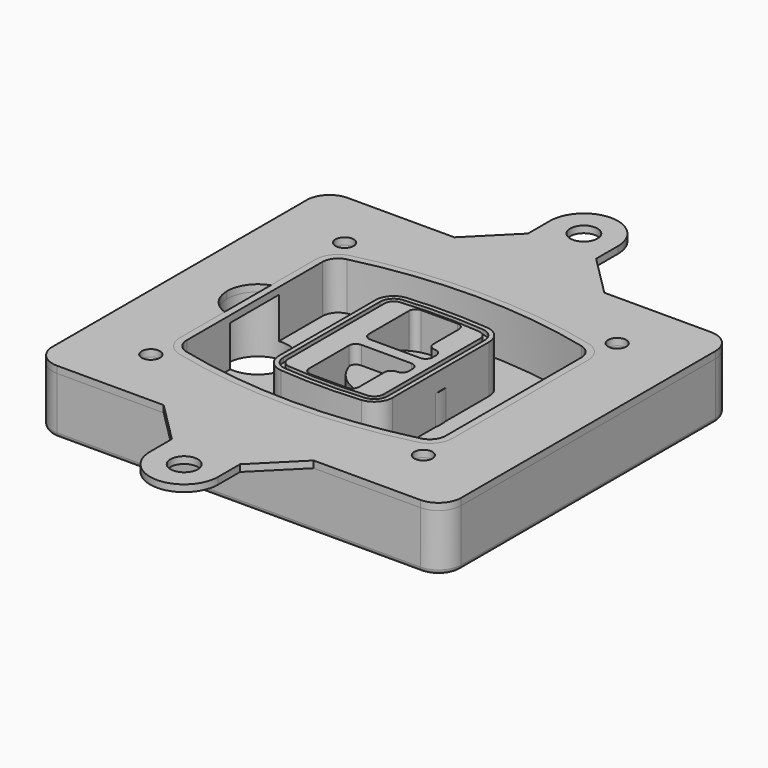
from build123d import *

# Parameters (mm, degrees)
F0_R      = 4
F1_DEPTH  = 25
F2_DEPTH  = 3
F3_DEPTH  = 18
F5_DEPTH  = 21
F6_DEPTH  = 2
F8_DEPTH  = 20
F9_DEPTH  = 16
F10_DEPTH = 25
F7_R      = 6
F7_R_2    = 4
F11_DEPTH = 6
F13_DEPTH = 9
F15_R     = 2
F16_R     = 6
F16_R_2   = 4
F17_DEPTH = 3


# Not quite as in the source:
# - a feature of the source that left no trace in its solid (it failed there, or was rolled back) is left out
# - a feature names something its author has since deleted; it is built from what else it names


with BuildPart() as f1:
    # F0 (on Top) → F1 (new body)
    with BuildSketch(Plane.XY):
        with BuildLine():
            ThreePointArc((-90, -70), (-87.0710678119, -77.0710678119), (-80, -80))
            Line((-80, -80), (80, -80))
            ThreePointArc((80, -80), (87.0710678119, -77.0710678119), (90, -70))
            Line((90, -70), (90, 70))
            ThreePointArc((90, 70), (87.0710678119, 77.0710678119), (80, 80))
            Line((80, 80), (-80, 80))
            ThreePointArc((-80, 80), (-87.0710678119, 77.0710678119), (-90, 70))
            Line((-90, 70), (-90, -70))
        make_face()
        with Locations((-60, -53.3333333333)):
            Circle(F0_R, mode=Mode.SUBTRACT)
        with Locations((60, -53.3333333333)):
            Circle(F0_R, mode=Mode.SUBTRACT)
        with Locations((-60, 53.3333333333)):
            Circle(F0_R, mode=Mode.SUBTRACT)
        with BuildLine():
            ThreePointArc((-64, 37.2990447398), (-61.0143011354, 45.9411029726), (-53.3306899286, 50.8970778549))
            ThreePointArc((-53.3306899286, 50.8970778549), (0, 57.3333333333), (53.3306899286, 50.8970778549))
            ThreePointArc((53.3306899286, 50.8970778549), (61.0143011354, 45.9411029726), (64, 37.2990447398))
            Line((64, 37.2990447398), (64, -37.2990447398))
            ThreePointArc((64, -37.2990447398), (61.0143011354, -45.9411029726), (53.3306899286, -50.8970778549))
            ThreePointArc((53.3306899286, -50.8970778549), (0, -57.3333333333), (-53.3306899286, -50.8970778549))
            ThreePointArc((-53.3306899286, -50.8970778549), (-61.0143011354, -45.9411029726), (-64, -37.2990447398))
            Line((-64, -37.2990447398), (-64, 37.2990447398))
        make_face(mode=Mode.SUBTRACT)
        with Locations((60, 53.3333333333)):
            Circle(F0_R, mode=Mode.SUBTRACT)
        with BuildLine():
            ThreePointArc((53.3306899286, 50.8970778549), (0, 57.3333333333), (-53.3306899286, 50.8970778549))
            ThreePointArc((-53.3306899286, 50.8970778549), (-61.0143011354, 45.9411029726), (-64, 37.2990447398))
            Line((-64, 37.2990447398), (-64, -37.2990447398))
            ThreePointArc((-64, -37.2990447398), (-61.0143011354, -45.9411029726), (-53.3306899286, -50.8970778549))
            ThreePointArc((-53.3306899286, -50.8970778549), (0, -57.3333333333), (53.3306899286, -50.8970778549))
            ThreePointArc((53.3306899286, -50.8970778549), (61.0143011354, -45.9411029726), (64, -37.2990447398))
            Line((64, -37.2990447398), (64, 37.2990447398))
            ThreePointArc((64, 37.2990447398), (61.0143011354, 45.9411029726), (53.3306899286, 50.8970778549))
        make_face()
        with BuildLine():
            Line((-60, -37.2990447398), (-60, 37.2990447398))
            ThreePointArc((-60, 37.2990447398), (-57.8673579538, 43.4719434775), (-52.3790642347, 47.0119255363))
            ThreePointArc((-52.3790642347, 47.0119255363), (0, 53.3333333333), (52.3790642347, 47.0119255363))
            ThreePointArc((52.3790642347, 47.0119255363), (57.8673579538, 43.4719434775), (60, 37.2990447398))
            Line((60, 37.2990447398), (60, -37.2990447398))
            ThreePointArc((60, -37.2990447398), (57.8673579538, -43.4719434775), (52.3790642347, -47.0119255363))
            ThreePointArc((52.3790642347, -47.0119255363), (0, -53.3333333333), (-52.3790642347, -47.0119255363))
            ThreePointArc((-52.3790642347, -47.0119255363), (-57.8673579538, -43.4719434775), (-60, -37.2990447398))
        make_face(mode=Mode.SUBTRACT)
        with BuildLine():
            ThreePointArc((-52.3790642347, 47.0119255363), (-57.8673579538, 43.4719434775), (-60, 37.2990447398))
            Line((-60, 37.2990447398), (-60, -37.2990447398))
            ThreePointArc((-60, -37.2990447398), (-57.8673579538, -43.4719434775), (-52.3790642347, -47.0119255363))
            ThreePointArc((-52.3790642347, -47.0119255363), (0, -53.3333333333), (52.3790642347, -47.0119255363))
            ThreePointArc((52.3790642347, -47.0119255363), (57.8673579538, -43.4719434775), (60, -37.2990447398))
            Line((60, -37.2990447398), (60, 37.2990447398))
            ThreePointArc((60, 37.2990447398), (57.8673579538, 43.4719434775), (52.3790642347, 47.0119255363))
            ThreePointArc((52.3790642347, 47.0119255363), (0, 53.3333333333), (-52.3790642347, 47.0119255363))
        make_face()
        with BuildLine():
            ThreePointArc((51.6653449643, 44.0980612973), (55.5071505677, 41.6200738562), (57, 37.2990447398))
            Line((57, 37.2990447398), (57, -37.2990447398))
            ThreePointArc((57, -37.2990447398), (55.5071505677, -41.6200738562), (51.6653449643, -44.0980612973))
            ThreePointArc((51.6653449643, -44.0980612973), (0, -50.3333333333), (-51.6653449643, -44.0980612973))
            ThreePointArc((-51.6653449643, -44.0980612973), (-55.5071505677, -41.6200738562), (-57, -37.2990447398))
            Line((-57, -37.2990447398), (-57, 37.2990447398))
            ThreePointArc((-57, 37.2990447398), (-55.5071505677, 41.6200738562), (-51.6653449643, 44.0980612973))
            ThreePointArc((-51.6653449643, 44.0980612973), (0, 50.3333333333), (51.6653449643, 44.0980612973))
        make_face(mode=Mode.SUBTRACT)
        with BuildLine():
            Line((57, -37.2990447398), (57, 37.2990447398))
            ThreePointArc((57, 37.2990447398), (55.5071505677, 41.6200738562), (51.6653449643, 44.0980612973))
            ThreePointArc((51.6653449643, 44.0980612973), (0, 50.3333333333), (-51.6653449643, 44.0980612973))
            ThreePointArc((-51.6653449643, 44.0980612973), (-55.5071505677, 41.6200738562), (-57, 37.2990447398))
            Line((-57, 37.2990447398), (-57, -37.2990447398))
            ThreePointArc((-57, -37.2990447398), (-55.5071505677, -41.6200738562), (-51.6653449643, -44.0980612973))
            ThreePointArc((-51.6653449643, -44.0980612973), (0, -50.3333333333), (51.6653449643, -44.0980612973))
            ThreePointArc((51.6653449643, -44.0980612973), (55.5071505677, -41.6200738562), (57, -37.2990447398))
        make_face()
    extrude(amount=-F1_DEPTH)

    # F0 (on Top) → F2 (join)
    with BuildSketch(Plane.XY):
        with BuildLine():
            ThreePointArc((-52.3790642347, 47.0119255363), (-57.8673579538, 43.4719434775), (-60, 37.2990447398))
            Line((-60, 37.2990447398), (-60, -37.2990447398))
            ThreePointArc((-60, -37.2990447398), (-57.8673579538, -43.4719434775), (-52.3790642347, -47.0119255363))
            ThreePointArc((-52.3790642347, -47.0119255363), (0, -53.3333333333), (52.3790642347, -47.0119255363))
            ThreePointArc((52.3790642347, -47.0119255363), (57.8673579538, -43.4719434775), (60, -37.2990447398))
            Line((60, -37.2990447398), (60, 37.2990447398))
            ThreePointArc((60, 37.2990447398), (57.8673579538, 43.4719434775), (52.3790642347, 47.0119255363))
            ThreePointArc((52.3790642347, 47.0119255363), (0, 53.3333333333), (-52.3790642347, 47.0119255363))
        make_face()
        with BuildLine():
            ThreePointArc((51.6653449643, 44.0980612973), (55.5071505677, 41.6200738562), (57, 37.2990447398))
            Line((57, 37.2990447398), (57, -37.2990447398))
            ThreePointArc((57, -37.2990447398), (55.5071505677, -41.6200738562), (51.6653449643, -44.0980612973))
            ThreePointArc((51.6653449643, -44.0980612973), (0, -50.3333333333), (-51.6653449643, -44.0980612973))
            ThreePointArc((-51.6653449643, -44.0980612973), (-55.5071505677, -41.6200738562), (-57, -37.2990447398))
            Line((-57, -37.2990447398), (-57, 37.2990447398))
            ThreePointArc((-57, 37.2990447398), (-55.5071505677, 41.6200738562), (-51.6653449643, 44.0980612973))
            ThreePointArc((-51.6653449643, 44.0980612973), (0, 50.3333333333), (51.6653449643, 44.0980612973))
        make_face(mode=Mode.SUBTRACT)
    extrude(amount=F2_DEPTH)

    # F0 (on Top) → F3 (cut)
    with BuildSketch(Plane.XY):
        with BuildLine():
            Line((57, -37.2990447398), (57, 37.2990447398))
            ThreePointArc((57, 37.2990447398), (55.5071505677, 41.6200738562), (51.6653449643, 44.0980612973))
            ThreePointArc((51.6653449643, 44.0980612973), (0, 50.3333333333), (-51.6653449643, 44.0980612973))
            ThreePointArc((-51.6653449643, 44.0980612973), (-55.5071505677, 41.6200738562), (-57, 37.2990447398))
            Line((-57, 37.2990447398), (-57, -37.2990447398))
            ThreePointArc((-57, -37.2990447398), (-55.5071505677, -41.6200738562), (-51.6653449643, -44.0980612973))
            ThreePointArc((-51.6653449643, -44.0980612973), (0, -50.3333333333), (51.6653449643, -44.0980612973))
            ThreePointArc((51.6653449643, -44.0980612973), (55.5071505677, -41.6200738562), (57, -37.2990447398))
        make_face()
    extrude(amount=-F3_DEPTH, mode=Mode.SUBTRACT)

    # F4 (on face) → F5 (join, through all)
    with BuildSketch(Plane.XY.offset(3)):
        with BuildLine():
            ThreePointArc((-25, -26.587695628), (-22.8992979869, -31.9912392117), (-17.7004291845, -34.5569740744))
            ThreePointArc((-17.7004291845, -34.5569740744), (0, -35.3333333333), (17.7004291845, -34.5569740744))
            ThreePointArc((17.7004291845, -34.5569740744), (22.8992979869, -31.9912392117), (25, -26.587695628))
            Line((25, -26.587695628), (25, 26.587695628))
            ThreePointArc((25, 26.587695628), (22.8992979869, 31.9912392117), (17.7004291845, 34.5569740744))
            ThreePointArc((17.7004291845, 34.5569740744), (0, 35.3333333333), (-17.7004291845, 34.5569740744))
            ThreePointArc((-17.7004291845, 34.5569740744), (-22.8992979869, 31.9912392117), (-25, 26.587695628))
            Line((-25, 26.587695628), (-25, -26.587695628))
        make_face()
        with BuildLine():
            ThreePointArc((17.5253218884, 32.5646544628), (21.4244734902, 30.6403533158), (23, 26.587695628))
            Line((23, 26.587695628), (23, -26.587695628))
            ThreePointArc((23, -26.587695628), (21.4244734902, -30.6403533158), (17.5253218884, -32.5646544628))
            ThreePointArc((17.5253218884, -32.5646544628), (0, -33.3333333333), (-17.5253218884, -32.5646544628))
            ThreePointArc((-17.5253218884, -32.5646544628), (-21.4244734902, -30.6403533158), (-23, -26.587695628))
            Line((-23, -26.587695628), (-23, 26.587695628))
            ThreePointArc((-23, 26.587695628), (-21.4244734902, 30.6403533158), (-17.5253218884, 32.5646544628))
            ThreePointArc((-17.5253218884, 32.5646544628), (0, 33.3333333333), (17.5253218884, 32.5646544628))
        make_face(mode=Mode.SUBTRACT)
        with BuildLine():
            Line((23, -26.587695628), (23, 26.587695628))
            ThreePointArc((23, 26.587695628), (21.4244734902, 30.6403533158), (17.5253218884, 32.5646544628))
            ThreePointArc((17.5253218884, 32.5646544628), (0, 33.3333333333), (-17.5253218884, 32.5646544628))
            ThreePointArc((-17.5253218884, 32.5646544628), (-21.4244734902, 30.6403533158), (-23, 26.587695628))
            Line((-23, 26.587695628), (-23, -26.587695628))
            ThreePointArc((-23, -26.587695628), (-21.4244734902, -30.6403533158), (-17.5253218884, -32.5646544628))
            ThreePointArc((-17.5253218884, -32.5646544628), (0, -33.3333333333), (17.5253218884, -32.5646544628))
            ThreePointArc((17.5253218884, -32.5646544628), (21.4244734902, -30.6403533158), (23, -26.587695628))
        make_face()
        with BuildLine():
            ThreePointArc((17.3502145923, 30.5723348512), (19.9496489934, 29.2894674198), (21, 26.587695628))
            Line((21, 26.587695628), (21, -26.587695628))
            ThreePointArc((21, -26.587695628), (19.9496489934, -29.2894674198), (17.3502145923, -30.5723348512))
            ThreePointArc((17.3502145923, -30.5723348512), (0, -31.3333333333), (-17.3502145923, -30.5723348512))
            ThreePointArc((-17.3502145923, -30.5723348512), (-19.9496489934, -29.2894674198), (-21, -26.587695628))
            Line((-21, -26.587695628), (-21, 26.587695628))
            ThreePointArc((-21, 26.587695628), (-19.9496489934, 29.2894674198), (-17.3502145923, 30.5723348512))
            ThreePointArc((-17.3502145923, 30.5723348512), (0, 31.3333333333), (17.3502145923, 30.5723348512))
        make_face(mode=Mode.SUBTRACT)
        with BuildLine():
            Line((21, -26.587695628), (21, 26.587695628))
            ThreePointArc((21, 26.587695628), (19.9496489934, 29.2894674198), (17.3502145923, 30.5723348512))
            ThreePointArc((17.3502145923, 30.5723348512), (0, 31.3333333333), (-17.3502145923, 30.5723348512))
            ThreePointArc((-17.3502145923, 30.5723348512), (-19.9496489934, 29.2894674198), (-21, 26.587695628))
            Line((-21, 26.587695628), (-21, -26.587695628))
            ThreePointArc((-21, -26.587695628), (-19.9496489934, -29.2894674198), (-17.3502145923, -30.5723348512))
            ThreePointArc((-17.3502145923, -30.5723348512), (0, -31.3333333333), (17.3502145923, -30.5723348512))
            ThreePointArc((17.3502145923, -30.5723348512), (19.9496489934, -29.2894674198), (21, -26.587695628))
        make_face()
        with BuildLine():
            Line((-8, -2.5), (14, -2.5))
            ThreePointArc((14, -2.5), (16.1213203436, -3.3786796564), (17, -5.5))
            Line((17, -5.5), (17, -7.5))
            ThreePointArc((17, -7.5), (16.1213203436, -9.6213203436), (14, -10.5))
            ThreePointArc((14, -10.5), (11.8786796564, -11.3786796564), (11, -13.5))
            Line((11, -13.5), (11, -27.5))
            ThreePointArc((11, -27.5), (10.1213203436, -29.6213203436), (8, -30.5))
            Line((8, -30.5), (-8, -30.5))
            ThreePointArc((-8, -30.5), (-10.1213203436, -29.6213203436), (-11, -27.5))
            Line((-11, -27.5), (-11, -5.5))
            ThreePointArc((-11, -5.5), (-10.1213203436, -3.3786796564), (-8, -2.5))
        make_face(mode=Mode.SUBTRACT)
        with BuildLine():
            ThreePointArc((-8, 2.5), (-10.1213203436, 3.3786796564), (-11, 5.5))
            Line((-11, 5.5), (-11, 27.5))
            ThreePointArc((-11, 27.5), (-10.1213203436, 29.6213203436), (-8, 30.5))
            Line((-8, 30.5), (8, 30.5))
            ThreePointArc((8, 30.5), (10.1213203436, 29.6213203436), (11, 27.5))
            Line((11, 27.5), (11, 13.5))
            ThreePointArc((11, 13.5), (11.8786796564, 11.3786796564), (14, 10.5))
            ThreePointArc((14, 10.5), (16.1213203436, 9.6213203436), (17, 7.5))
            Line((17, 7.5), (17, 5.5))
            ThreePointArc((17, 5.5), (16.1213203436, 3.3786796564), (14, 2.5))
            Line((14, 2.5), (-8, 2.5))
        make_face(mode=Mode.SUBTRACT)
    extrude(amount=-F5_DEPTH)

    # F4 (on face) → F6 (cut)
    with BuildSketch(Plane.XY.offset(3)):
        with BuildLine():
            Line((23, -26.587695628), (23, 26.587695628))
            ThreePointArc((23, 26.587695628), (21.4244734902, 30.6403533158), (17.5253218884, 32.5646544628))
            ThreePointArc((17.5253218884, 32.5646544628), (0, 33.3333333333), (-17.5253218884, 32.5646544628))
            ThreePointArc((-17.5253218884, 32.5646544628), (-21.4244734902, 30.6403533158), (-23, 26.587695628))
            Line((-23, 26.587695628), (-23, -26.587695628))
            ThreePointArc((-23, -26.587695628), (-21.4244734902, -30.6403533158), (-17.5253218884, -32.5646544628))
            ThreePointArc((-17.5253218884, -32.5646544628), (0, -33.3333333333), (17.5253218884, -32.5646544628))
            ThreePointArc((17.5253218884, -32.5646544628), (21.4244734902, -30.6403533158), (23, -26.587695628))
        make_face()
        with BuildLine():
            ThreePointArc((17.3502145923, 30.5723348512), (19.9496489934, 29.2894674198), (21, 26.587695628))
            Line((21, 26.587695628), (21, -26.587695628))
            ThreePointArc((21, -26.587695628), (19.9496489934, -29.2894674198), (17.3502145923, -30.5723348512))
            ThreePointArc((17.3502145923, -30.5723348512), (0, -31.3333333333), (-17.3502145923, -30.5723348512))
            ThreePointArc((-17.3502145923, -30.5723348512), (-19.9496489934, -29.2894674198), (-21, -26.587695628))
            Line((-21, -26.587695628), (-21, 26.587695628))
            ThreePointArc((-21, 26.587695628), (-19.9496489934, 29.2894674198), (-17.3502145923, 30.5723348512))
            ThreePointArc((-17.3502145923, 30.5723348512), (0, 31.3333333333), (17.3502145923, 30.5723348512))
        make_face(mode=Mode.SUBTRACT)
    extrude(amount=-F6_DEPTH, mode=Mode.SUBTRACT)

    # F7 (on face) → F8 (join)
    with BuildSketch(Plane(origin=(0, 0, -25), x_dir=(1, 0, 0), z_dir=(0, 0, -1))):
        with BuildLine():
            ThreePointArc((-6.71157564, 0), (6.7567035675, 13.4682792075), (20.224982775, 0))
            Line((20.224982775, 0), (25.224982775, 0))
            ThreePointArc((25.224982775, 0), (6.7567035675, 18.4682792075), (-11.71157564, 0))
            Line((-11.71157564, 0), (-6.71157564, 0))
        make_face()
        with BuildLine():
            Line((-6.71157564, 0), (20.224982775, 0))
            ThreePointArc((20.224982775, 0), (6.7567035675, 13.4682792075), (-6.71157564, 0))
        make_face()
        with BuildLine():
            ThreePointArc((-6.71157564, 0), (6.7567035675, -13.4682792075), (20.224982775, 0))
            Line((20.224982775, 0), (-6.71157564, 0))
        make_face()
        with BuildLine():
            Line((25.224982775, 0), (20.224982775, 0))
            ThreePointArc((20.224982775, 0), (6.7567035675, -13.4682792075), (-6.71157564, 0))
            Line((-6.71157564, 0), (-11.71157564, 0))
            ThreePointArc((-11.71157564, 0), (6.7567035675, -18.4682792075), (25.224982775, 0))
        make_face()
    extrude(amount=-F8_DEPTH)

    # F7 (on face) → F9 (cut)
    with BuildSketch(Plane(origin=(0, 0, -25), x_dir=(1, 0, 0), z_dir=(0, 0, -1))):
        with BuildLine():
            Line((-6.71157564, 0), (20.224982775, 0))
            ThreePointArc((20.224982775, 0), (6.7567035675, 13.4682792075), (-6.71157564, 0))
        make_face()
        with BuildLine():
            ThreePointArc((-6.71157564, 0), (6.7567035675, -13.4682792075), (20.224982775, 0))
            Line((20.224982775, 0), (-6.71157564, 0))
        make_face()
    extrude(amount=-F9_DEPTH, mode=Mode.SUBTRACT)

    # F7 (on face) → F10 (cut)
    with BuildSketch(Plane(origin=(0, 0, -25), x_dir=(1, 0, 0), z_dir=(0, 0, -1))):
        with BuildLine():
            Line((-69.0318229325, 0), (-42.0952645175, 0))
            ThreePointArc((-42.0952645175, 0), (-55.563543725, 13.4682792075), (-69.0318229325, 0))
        make_face()
        with BuildLine():
            ThreePointArc((-69.0318229325, 0), (-55.563543725, -13.4682792075), (-42.0952645175, 0))
            Line((-42.0952645175, 0), (-69.0318229325, 0))
        make_face()
    extrude(amount=-F10_DEPTH, mode=Mode.SUBTRACT)

    # F7 (on face) → F11 (cut)
    with BuildSketch(Plane(origin=(0, 0, -25), x_dir=(1, 0, 0), z_dir=(0, 0, -1))):
        with Locations((60, -53.3333333333)):
            Circle(F7_R)
        with Locations((60, -53.3333333333)):
            Circle(F7_R_2, mode=Mode.SUBTRACT)
        with Locations((-60, -53.3333333333)):
            Circle(F7_R)
        with Locations((-60, -53.3333333333)):
            Circle(F7_R_2, mode=Mode.SUBTRACT)
        with Locations((-60, 53.3333333333)):
            Circle(F7_R)
        with Locations((-60, 53.3333333333)):
            Circle(F7_R_2, mode=Mode.SUBTRACT)
        with Locations((60, 53.3333333333)):
            Circle(F7_R)
        with Locations((60, 53.3333333333)):
            Circle(F7_R_2, mode=Mode.SUBTRACT)
    extrude(amount=-F11_DEPTH, mode=Mode.SUBTRACT)

    # F12 (on face) → F13 (cut, through all)
    with BuildSketch(Plane(origin=(0, 0, -9), x_dir=(1, 0, 0), z_dir=(0, 0, -1))):
        with BuildLine():
            ThreePointArc((20.224982775, 0), (20.1663399806, 1.2554664788), (19.9909222755, 2.5))
            Line((19.9909222755, 2.5), (14, 2.5))
            ThreePointArc((14, 2.5), (16.1213203436, 3.3786796564), (17, 5.5))
            Line((17, 5.5), (17, 7.5))
            ThreePointArc((17, 7.5), (16.1213203436, 9.6213203436), (14, 10.5))
            ThreePointArc((14, 10.5), (12.1627255951, 11.1284134507), (11.0951631559, 12.750384826))
            ThreePointArc((11.0951631559, 12.750384826), (11.0476113807, 12.7664660322), (11, 12.7823698976))
            Line((11, 12.7823698976), (11, -12.7823698976))
            ThreePointArc((11, -12.7823698976), (11.0476113807, -12.7664660322), (11.0951631559, -12.750384826))
            ThreePointArc((11.0951631559, -12.750384826), (12.1627255951, -11.1284134507), (14, -10.5))
            ThreePointArc((14, -10.5), (16.1213203436, -9.6213203436), (17, -7.5))
            Line((17, -7.5), (17, -5.5))
            ThreePointArc((17, -5.5), (16.1213203436, -3.3786796564), (14, -2.5))
            Line((14, -2.5), (19.9909222755, -2.5))
            ThreePointArc((19.9909222755, -2.5), (20.1663399806, -1.2554664788), (20.224982775, 0))
        make_face()
    extrude(amount=F13_DEPTH, mode=Mode.SUBTRACT)

    # F15
    f15_edges = [f1.edges().sort_by_distance(p)[0] for p in [
        (0, -80, -25),
        (-87.071068, -77.071068, -25),
        (-90, 0, -25),
        (-87.071068, 77.071068, -25),
        (87.071068, -77.071068, -25),
        (0, 80, -25),
        (90, 0, -25),
        (87.071068, 77.071068, -25),
    ]]
    fillet(f15_edges, radius=F15_R)


with BuildPart() as f17:
    # F16 (on face) → F17 (new body, through all)
    with BuildSketch(Plane.XY):
        with BuildLine():
            Line((-15, 98), (-33, 80))
            Line((-33, 80), (33, 80))
            Line((33, 80), (15, 98))
            Line((15, 98), (15, 110))
            ThreePointArc((15, 110), (0, 125), (-15, 110))
            Line((-15, 110), (-15, 98))
        make_face()
        with Locations((0, 110)):
            Circle(F16_R, mode=Mode.SUBTRACT)
        with BuildLine():
            Line((33, -80), (-33, -80))
            Line((-33, -80), (-15, -98))
            Line((-15, -98), (-15, -110))
            ThreePointArc((-15, -110), (0, -125), (15, -110))
            Line((15, -110), (15, -98))
            Line((15, -98), (33, -80))
        make_face()
        with Locations((0, -110)):
            Circle(F16_R, mode=Mode.SUBTRACT)
        with BuildLine():
            Line((33, 80), (-33, 80))
            Line((-33, 80), (-80, 80))
            ThreePointArc((-80, 80), (-87.0710678119, 77.0710678119), (-90, 70))
            Line((-90, 70), (-90, -70))
            ThreePointArc((-90, -70), (-87.0710678119, -77.0710678119), (-80, -80))
            Line((-80, -80), (-33, -80))
            Line((-33, -80), (33, -80))
            Line((33, -80), (80, -80))
            ThreePointArc((80, -80), (87.0710678119, -77.0710678119), (90, -70))
            Line((90, -70), (90, 70))
            ThreePointArc((90, 70), (87.0710678119, 77.0710678119), (80, 80))
            Line((80, 80), (33, 80))
        make_face()
        with Locations((-60, -53.3333333333)):
            Circle(F16_R_2, mode=Mode.SUBTRACT)
        with BuildLine():
            Line((-60, 12.7166190685), (-60, 37.2990447398))
            ThreePointArc((-60, 37.2990447398), (-57.8673579538, 43.4719434775), (-52.3790642347, 47.0119255363))
            ThreePointArc((-52.3790642347, 47.0119255363), (0, 53.3333333333), (52.3790642347, 47.0119255363))
            ThreePointArc((52.3790642347, 47.0119255363), (57.8673579538, 43.4719434775), (60, 37.2990447398))
            Line((60, 37.2990447398), (60, -37.2990447398))
            ThreePointArc((60, -37.2990447398), (57.8673579538, -43.4719434775), (52.3790642347, -47.0119255363))
            ThreePointArc((52.3790642347, -47.0119255363), (0, -53.3333333333), (-52.3790642347, -47.0119255363))
            ThreePointArc((-52.3790642347, -47.0119255363), (-57.8673579538, -43.4719434775), (-60, -37.2990447398))
            Line((-60, -37.2990447398), (-60, -12.7166190685))
            ThreePointArc((-60, -12.7166190685), (-66.5441169481, -7.798817635), (-69.0318229325, 0))
            ThreePointArc((-69.0318229325, 0), (-66.5441169481, 7.798817635), (-60, 12.7166190685))
        make_face(mode=Mode.SUBTRACT)
        with Locations((60, -53.3333333333)):
            Circle(F16_R_2, mode=Mode.SUBTRACT)
        with Locations((-60, 53.3333333333)):
            Circle(F16_R_2, mode=Mode.SUBTRACT)
        with Locations((60, 53.3333333333)):
            Circle(F16_R_2, mode=Mode.SUBTRACT)
    extrude(amount=F17_DEPTH)


solid = Compound([f1.part, f17.part])
